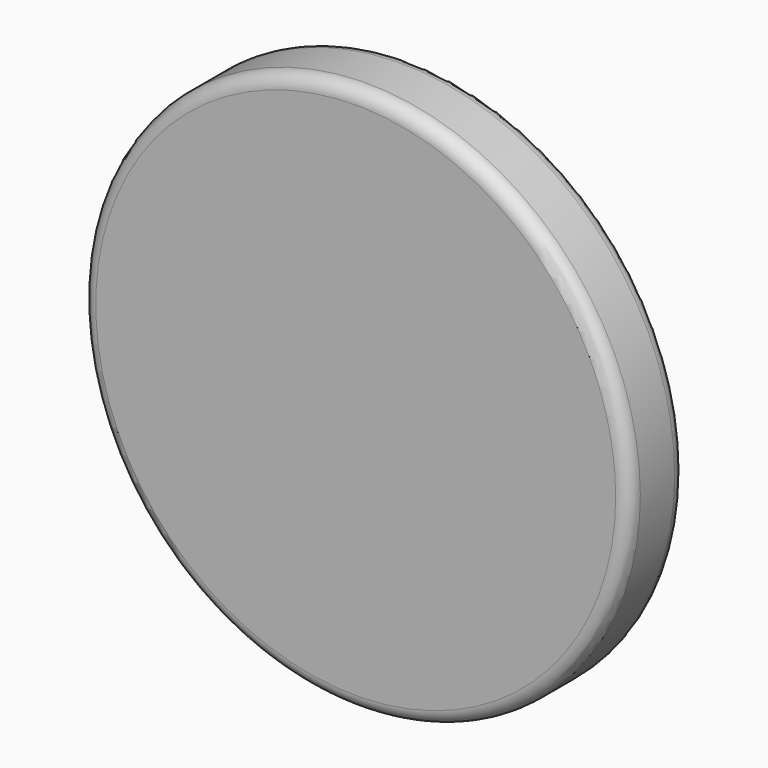
from build123d import *

# Parameters (mm, degrees)
F0_R     = 101.6
F1_DEPTH = 25.4
F2_T     = -2.54


# Not quite as in the source:
# - a fillet or chamfer that OpenCascade refuses, or shapes differently, is made with other operations: its cross-section is extruded or revolved along the edge and cut away or added


with BuildPart() as f1:
    # F0 (on Front) → F1 (new body)
    with BuildSketch(Plane.XZ):
        Circle(F0_R)
    extrude(amount=F1_DEPTH)

    # F2
    f2_openings = [f1.faces().sort_by_distance(p)[0] for p in [
        (0, 0, 0),
    ]]
    offset(amount=F2_T, openings=f2_openings)

    # F3: fillet of radius 5.08 on 2 edges, made by hand

    # F3_s1 → F3_t2 (revolve, cut)
    with BuildSketch(Plane.XY):
        with BuildLine():
            ThreePointArc((101.6, -20.32), (100.1121024484, -23.9121024484), (96.52, -25.4))
            Line((96.52, -25.4), (101.6, -25.4))
            Line((101.6, -25.4), (101.6, -20.32))
        make_face()
    revolve(axis=Axis((0, -25.4, 0), (0, -1, 0)), mode=Mode.SUBTRACT)

    # F3_s3 → F3_t4 (revolve, cut)
    with BuildSketch(Plane.XY):
        with BuildLine():
            ThreePointArc((101.6, -4.3994090512), (100.9194090512, -1.8594090512), (99.06, 0))
            Line((99.06, 0), (101.6, 0))
            Line((101.6, 0), (101.6, -4.3994090512))
        make_face()
    revolve(axis=Axis((0, 0, 0), (0, -1, 0)), mode=Mode.SUBTRACT)


solid = f1.part
